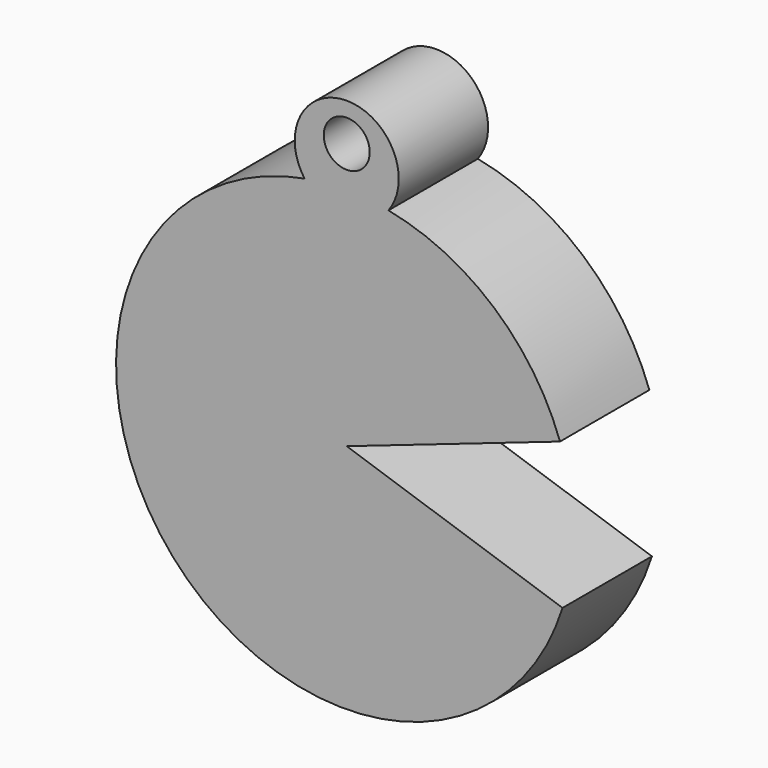
from build123d import *

# Parameters (mm, degrees)
F0_R     = 5.227515474
F1_DEPTH = 25.4
F2_DEPTH = 25.4


# Not quite as in the source:
# - a feature names something its author has since deleted; it is built from what else it names


with BuildPart() as f1:
    # F0 (on Front) → F1 (new body)
    with BuildSketch(Plane.XZ):
        with BuildLine():
            Line((0, 0), (48.4997071326, 16.699001193))
            ThreePointArc((48.4997071326, 16.699001193), (33.4463476719, 38.6685413288), (9.4887581342, 50.3003179933))
            ThreePointArc((9.4887581342, 50.3003179933), (0.0976286062, 69.1824149389), (-9.603985867, 50.457950314))
            ThreePointArc((-9.603985867, 50.457950314), (-39.5504687593, -35.0093012615), (49.08054322, -16.408585012))
            Line((49.08054322, -16.408585012), (0, 0))
        make_face()
        with Locations((0, 60.5520345271)):
            Circle(F0_R, mode=Mode.SUBTRACT)
    extrude(amount=F1_DEPTH)

    # F0 (on Front) → F2 (join)
    with BuildSketch(Plane.XZ):
        with BuildLine():
            Line((0, 0), (48.4997071326, 16.699001193))
            ThreePointArc((48.4997071326, 16.699001193), (33.4463476719, 38.6685413288), (9.4887581342, 50.3003179933))
            ThreePointArc((9.4887581342, 50.3003179933), (0.0976286062, 69.1824149389), (-9.603985867, 50.457950314))
            ThreePointArc((-9.603985867, 50.457950314), (-39.5504687593, -35.0093012615), (49.08054322, -16.408585012))
            Line((49.08054322, -16.408585012), (0, 0))
        make_face()
        with Locations((0, 60.5520345271)):
            Circle(F0_R, mode=Mode.SUBTRACT)
    extrude(amount=F2_DEPTH)


solid = f1.part
